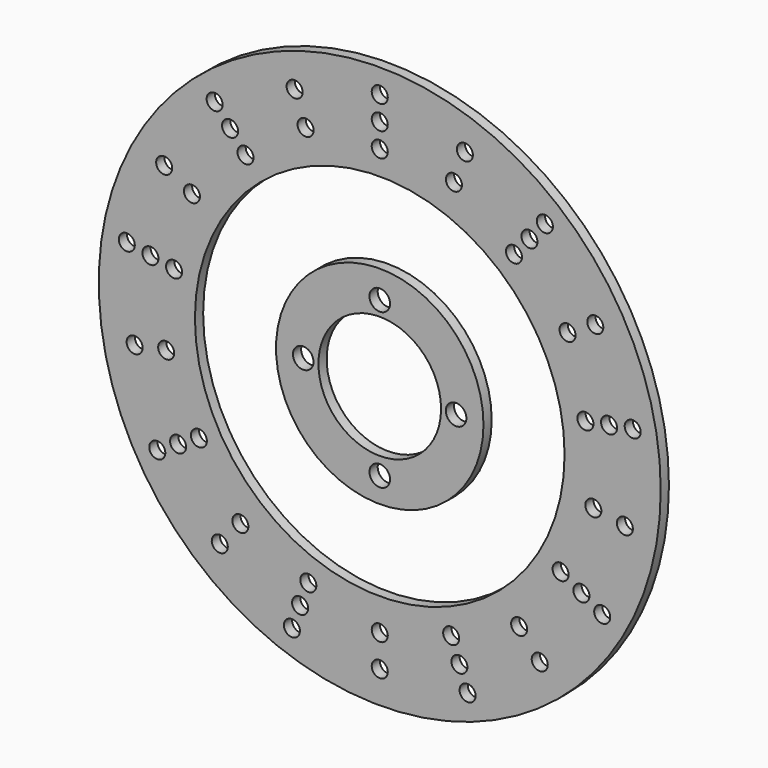
from build123d import *

# Parameters (mm, degrees)
F0_R            = 138.811
F0_R_2          = 91.313
F3_DEPTH        = 5.08
F2_R            = 3.9624
F4_DEPTH        = 5.081
F4_COPIES_COUNT = 9
F6_D            = 7.9248
F6_COPIES_COUNT = 9
F0_R_3          = 51.2445
F0_R_4          = 30.2895
F7_DEPTH        = 5.08
F8_D            = 10.16


# Not quite as in the source:
# - a pattern or mirror of a feature is missing from the dataset's text; its kind, count and spacing are read off the source's solid


with BuildPart() as f3:
    # F0 (on Front) → F3 (new body)
    with BuildSketch(Plane.XZ):
        Circle(F0_R)
        Circle(F0_R_2, mode=Mode.SUBTRACT)
    extrude(amount=F3_DEPTH)

    # F2 (on face) → F4 (cut, through all)
    with BuildSketch(Plane.XZ):
        with Locations((0, 103.1748)):
            Circle(F2_R)
        with Locations((0, 115.0366)):
            Circle(F2_R)
        with Locations((0, 126.8984)):
            Circle(F2_R)
    f4 = extrude(amount=F4_DEPTH, mode=Mode.SUBTRACT)

    # F4_copies: F4 ×9 about axis
    f4_copies_axis = Axis((0, 0, 0), (0, 1, 0))
    for i in range(1, F4_COPIES_COUNT):
        add(f4.rotate(f4_copies_axis, i * 360 / F4_COPIES_COUNT), mode=Mode.SUBTRACT)

    # F6 (through all)
    with Locations(Plane(origin=(0, 0, 0), x_dir=(1, 0, 0), z_dir=(0, 1, 0))):
        with Locations((0, 107.1372), (0, 122.9614)):
            f6 = Hole(F6_D / 2)

    # F6_copies: F6 ×9 about axis
    f6_copies_axis = Axis((0, 0, 0), (0, 1, 0))
    for i in range(1, F6_COPIES_COUNT):
        add(f6.rotate(f6_copies_axis, i * 360 / F6_COPIES_COUNT), mode=Mode.SUBTRACT)


with BuildPart() as f7:
    # F0 (on Front) → F7 (new body)
    with BuildSketch(Plane.XZ):
        Circle(F0_R_3)
        Circle(F0_R_4, mode=Mode.SUBTRACT)
    extrude(amount=F7_DEPTH)

    # F8 (through all)
    with Locations(Plane(origin=(0, 0, 0), x_dir=(1, 0, 0), z_dir=(0, 1, 0))):
        with Locations((0, -37.5412), (37.7119863628, 0), (0, 38.8407654956), (-37.8069085799, 0)):
            Hole(F8_D / 2)


solid = Compound([f3.part, f7.part])
